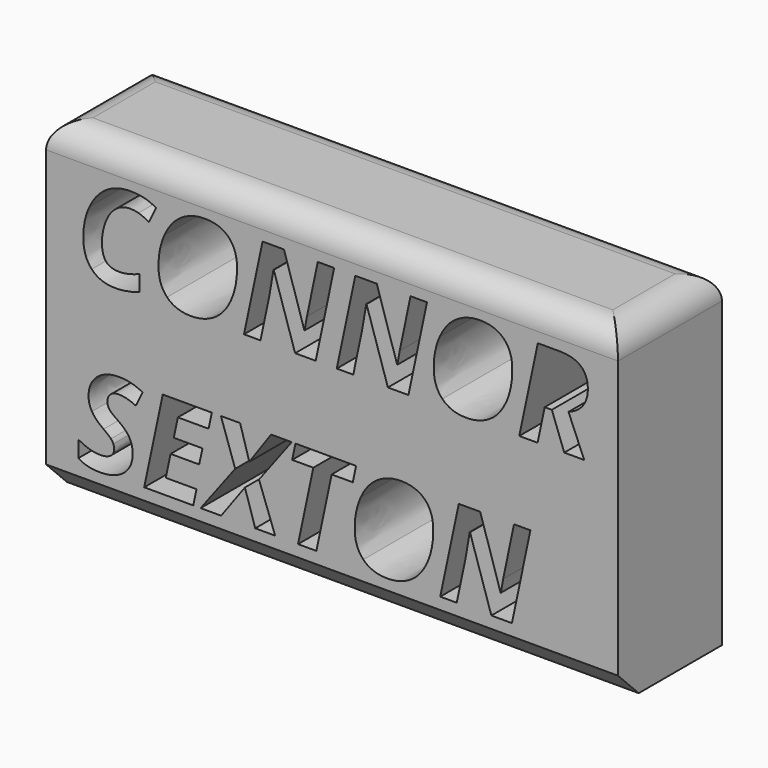
from build123d import *

# Parameters (mm, degrees)
F0_W     = 111.7530614138
F0_H     = 64.2868950963
F1_DEPTH = 25.4
F2_R     = 5.08
F3_SIZE  = 5.08


with BuildPart() as f1:
    # F0 (on Front) → F1 (new body)
    with BuildSketch(Plane.XZ):
        with Locations((-55.8765307069, 32.1434475482)):
            Rectangle(F0_W, F0_H)
        with BuildLine():
            add(Edge.make_bspline(
                [(-95.5342243518, 15.0884542018), (-94.8306232438, 13.9570636201), (-94.8306232438, 12.4447903053)],
                knots=[0, 0, 0, 1, 1, 1], degree=2))
            add(Edge.make_bspline(
                [(-94.8306232438, 12.4447903053), (-94.8306232438, 9.9943821797), (-96.5661726436, 8.5684172674)],
                knots=[0, 0, 0, 1, 1, 1], degree=2))
            add(Edge.make_bspline(
                [(-96.5661726436, 8.5684172674), (-98.3017220434, 7.1424523551), (-101.2662280453, 7.1424523551)],
                knots=[0, 0, 0, 1, 1, 1], degree=2))
            add(Edge.make_bspline(
                [(-101.2662280453, 7.1424523551), (-103.8592326621, 7.1424523551), (-105.4428042226, 8.2006684216)],
                knots=[0, 0, 0, 1, 1, 1], degree=2))
            Line((-105.4428042226, 8.2006684216), (-105.4428042226, 11.4128420135))
            add(Edge.make_bspline(
                [(-105.4428042226, 11.4128420135), (-103.1800230591, 10.1482362886), (-101.2437128098, 10.1482362886)],
                knots=[0, 0, 0, 1, 1, 1], degree=2))
            add(Edge.make_bspline(
                [(-101.2437128098, 10.1482362886), (-99.9303240748, 10.1482362886), (-99.191073844, 10.6454477383)],
                knots=[0, 0, 0, 1, 1, 1], degree=2))
            add(Edge.make_bspline(
                [(-99.191073844, 10.6454477383), (-98.4518236131, 11.142659188), (-98.4518236131, 12.0094957531)],
                knots=[0, 0, 0, 1, 1, 1], degree=2))
            add(Edge.make_bspline(
                [(-98.4518236131, 12.0094957531), (-98.4518236131, 12.5160885509), (-98.611306531, 12.896971284)],
                knots=[0, 0, 0, 1, 1, 1], degree=2))
            add(Edge.make_bspline(
                [(-98.611306531, 12.896971284), (-98.7707894488, 13.2778540172), (-99.0634875097, 13.6062012009)],
                knots=[0, 0, 0, 1, 1, 1], degree=2))
            add(Edge.make_bspline(
                [(-99.0634875097, 13.6062012009), (-99.3561855707, 13.9345483847), (-100.5157201967, 14.8013849498)],
                knots=[0, 0, 0, 1, 1, 1], degree=2))
            add(Edge.make_bspline(
                [(-100.5157201967, 14.8013849498), (-102.1368171496, 15.9646721151), (-102.7935115171, 17.1016915056)],
                knots=[0, 0, 0, 1, 1, 1], degree=2))
            add(Edge.make_bspline(
                [(-102.7935115171, 17.1016915056), (-103.4502058846, 18.2387108962), (-103.4502058846, 19.5520996312)],
                knots=[0, 0, 0, 1, 1, 1], degree=2))
            add(Edge.make_bspline(
                [(-103.4502058846, 19.5520996312), (-103.4502058846, 21.0643729461), (-102.7222132715, 22.2539278861)],
                knots=[0, 0, 0, 1, 1, 1], degree=2))
            add(Edge.make_bspline(
                [(-102.7222132715, 22.2539278861), (-101.9942206584, 23.443482826), (-100.6508116094, 24.1058060024)],
                knots=[0, 0, 0, 1, 1, 1], degree=2))
            add(Edge.make_bspline(
                [(-100.6508116094, 24.1058060024), (-99.3074025605, 24.7681291788), (-97.5624718126, 24.7681291788)],
                knots=[0, 0, 0, 1, 1, 1], degree=2))
            add(Edge.make_bspline(
                [(-97.5624718126, 24.7681291788), (-95.0182502059, 24.7681291788), (-92.9055706122, 23.6085945527)],
                knots=[0, 0, 0, 1, 1, 1], degree=2))
            Line((-92.9055706122, 23.6085945527), (-94.185186494, 20.8767459839))
            add(Edge.make_bspline(
                [(-94.185186494, 20.8767459839), (-96.0126731053, 21.743582549), (-97.5624718126, 21.743582549)],
                knots=[0, 0, 0, 1, 1, 1], degree=2))
            add(Edge.make_bspline(
                [(-97.5624718126, 21.743582549), (-98.5343794765, 21.743582549), (-99.1554247212, 21.2163507854)],
                knots=[0, 0, 0, 1, 1, 1], degree=2))
            add(Edge.make_bspline(
                [(-99.1554247212, 21.2163507854), (-99.7764699659, 20.6891190218), (-99.7764699659, 19.8222824567)],
                knots=[0, 0, 0, 1, 1, 1], degree=2))
            add(Edge.make_bspline(
                [(-99.7764699659, 19.8222824567), (-99.7764699659, 19.1055474613), (-99.3899584238, 18.5726868888)],
                knots=[0, 0, 0, 1, 1, 1], degree=2))
            add(Edge.make_bspline(
                [(-99.3899584238, 18.5726868888), (-99.0034468818, 18.0398263163), (-97.6562852937, 17.1579795943)],
                knots=[0, 0, 0, 1, 1, 1], degree=2))
            add(Edge.make_bspline(
                [(-97.6562852937, 17.1579795943), (-96.2378254599, 16.2198447836), (-95.5342243518, 15.0884542018)],
                knots=[0, 0, 0, 1, 1, 1], degree=2))
        make_face(mode=Mode.SUBTRACT)
        Polygon((-82.3609353398, 10.3808937217), (-82.9951144719, 7.3788623274), (-92.5753471588, 7.3788623274), (-88.9541467895, 24.524214128), (-79.3589039455, 24.524214128), (-79.9930830776, 21.5446979692), (-85.9971458661, 21.5446979692), (-86.7851791071, 17.7809011086), (-81.1901430961, 17.7809011086), (-81.8355798458, 14.8013849498), (-87.4268633177, 14.8013849498), (-88.3649981284, 10.3808937217), align=None, mode=Mode.SUBTRACT)
        Polygon((-70.1426675651, 16.0209602037), (-66.9980396796, 7.3788623274), (-70.881917796, 7.3788623274), (-72.8970313694, 13.7469214225), (-77.542674952, 7.3788623274), (-81.5541394026, 7.3788623274), (-74.7995687655, 16.3399260393), (-77.5877054229, 24.524214128), (-73.8351661801, 24.524214128), (-72.041452422, 18.4488530938), (-67.7860729206, 24.524214128), (-63.7520932346, 24.524214128), align=None, mode=Mode.SUBTRACT)
        Polygon((-55.9543166879, 21.4996674982), (-58.9338328467, 7.3788623274), (-62.5100027452, 7.3788623274), (-59.5304865864, 21.4996674982), (-63.6582797535, 21.4996674982), (-63.0128430037, 24.524214128), (-51.1698291533, 24.524214128), (-51.8152659031, 21.4996674982), align=None, mode=Mode.SUBTRACT)
        with BuildLine():
            add(Edge.make_bspline(
                [(-37.7301098551, 23.1057542942), (-36.0883739363, 21.4171116349), (-36.0883739363, 18.3775548482)],
                knots=[0, 0, 0, 1, 1, 1], degree=2))
            add(Edge.make_bspline(
                [(-36.0883739363, 18.3775548482), (-36.0883739363, 15.0603101575), (-37.249784832, 12.4391614964)],
                knots=[0, 0, 0, 1, 1, 1], degree=2))
            add(Edge.make_bspline(
                [(-37.249784832, 12.4391614964), (-38.4111957276, 9.8180128353), (-40.4281855707, 8.4802325952)],
                knots=[0, 0, 0, 1, 1, 1], degree=2))
            add(Edge.make_bspline(
                [(-40.4281855707, 8.4802325952), (-42.4451754137, 7.1424523551), (-45.0719528837, 7.1424523551)],
                knots=[0, 0, 0, 1, 1, 1], degree=2))
            add(Edge.make_bspline(
                [(-45.0719528837, 7.1424523551), (-48.073984278, 7.1424523551), (-49.7569981284, 8.8723729461)],
                knots=[0, 0, 0, 1, 1, 1], degree=2))
            add(Edge.make_bspline(
                [(-49.7569981284, 8.8723729461), (-51.4400119788, 10.602293537), (-51.4400119788, 13.6756231769)],
                knots=[0, 0, 0, 1, 1, 1], degree=2))
            add(Edge.make_bspline(
                [(-51.4400119788, 13.6756231769), (-51.4400119788, 16.78272567), (-50.2786010831, 19.3926167134)],
                knots=[0, 0, 0, 1, 1, 1], degree=2))
            add(Edge.make_bspline(
                [(-50.2786010831, 19.3926167134), (-49.1171901875, 22.0025077568), (-47.0758088394, 23.3984523551)],
                knots=[0, 0, 0, 1, 1, 1], degree=2))
            add(Edge.make_bspline(
                [(-47.0758088394, 23.3984523551), (-45.0344274913, 24.7943969535), (-42.3626195503, 24.7943969535)],
                knots=[0, 0, 0, 1, 1, 1], degree=2))
            add(Edge.make_bspline(
                [(-42.3626195503, 24.7943969535), (-39.3718457738, 24.7943969535), (-37.7301098551, 23.1057542942)],
                knots=[0, 0, 0, 1, 1, 1], degree=2))
        make_face(mode=Mode.SUBTRACT)
        with BuildLine():
            Line((-17.1005253675, 24.524214128), (-20.7254782761, 7.3788623274))
            Line((-20.7254782761, 7.3788623274), (-24.7369427267, 7.3788623274))
            Line((-24.7369427267, 7.3788623274), (-28.9097663648, 20.3476379507))
            Line((-28.9097663648, 20.3476379507), (-28.9810646104, 20.3476379507))
            Line((-28.9810646104, 20.3476379507), (-29.0298476205, 19.9723840264))
            add(Edge.make_bspline(
                [(-29.0298476205, 19.9723840264), (-29.4051015448, 17.4394200375), (-29.8028707045, 15.4468216995)],
                knots=[0, 0, 0, 1, 1, 1], degree=2))
            Line((-29.8028707045, 15.4468216995), (-31.5027709816, 7.3788623274))
            Line((-31.5027709816, 7.3788623274), (-34.7262021912, 7.3788623274))
            Line((-34.7262021912, 7.3788623274), (-31.1050018218, 24.524214128))
            Line((-31.1050018218, 24.524214128), (-26.9171680268, 24.524214128))
            Line((-26.9171680268, 24.524214128), (-22.9319713509, 11.8931670366))
            Line((-22.9319713509, 11.8931670366), (-22.8831883407, 11.8931670366))
            add(Edge.make_bspline(
                [(-22.8831883407, 11.8931670366), (-22.7443443888, 12.7862713764), (-22.4272548227, 14.4392649128)],
                knots=[0, 0, 0, 1, 1, 1], degree=2))
            add(Edge.make_bspline(
                [(-22.4272548227, 14.4392649128), (-22.1101652567, 16.0922584493), (-20.3164514986, 24.524214128)],
                knots=[0, 0, 0, 1, 1, 1], degree=2))
            Line((-20.3164514986, 24.524214128), (-17.1005253675, 24.524214128))
        make_face(mode=Mode.SUBTRACT)
        with BuildLine():
            add(Edge.make_bspline(
                [(-93.7029852013, 54.2067995389), (-94.5116574081, 54.4281993542), (-95.3109482669, 54.4281993542)],
                knots=[0, 0, 0, 1, 1, 1], degree=2))
            add(Edge.make_bspline(
                [(-95.3109482669, 54.4281993542), (-96.8569944349, 54.4281993542), (-98.0953323851, 53.4788069258)],
                knots=[0, 0, 0, 1, 1, 1], degree=2))
            add(Edge.make_bspline(
                [(-98.0953323851, 53.4788069258), (-99.3336703352, 52.5294144973), (-100.0841781838, 50.6831651898)],
                knots=[0, 0, 0, 1, 1, 1], degree=2))
            add(Edge.make_bspline(
                [(-100.0841781838, 50.6831651898), (-100.8346860323, 48.8369158824), (-100.8346860323, 46.7129786709)],
                knots=[0, 0, 0, 1, 1, 1], degree=2))
            add(Edge.make_bspline(
                [(-100.8346860323, 46.7129786709), (-100.8346860323, 44.7541531862), (-100.0316426344, 43.8047607577)],
                knots=[0, 0, 0, 1, 1, 1], degree=2))
            add(Edge.make_bspline(
                [(-100.0316426344, 43.8047607577), (-99.2285992364, 42.8553683293), (-97.4686583315, 42.8553683293)],
                knots=[0, 0, 0, 1, 1, 1], degree=2))
            add(Edge.make_bspline(
                [(-97.4686583315, 42.8553683293), (-95.7575004368, 42.8553683293), (-93.5059768911, 43.7597302868)],
                knots=[0, 0, 0, 1, 1, 1], degree=2))
            Line((-93.5059768911, 43.7597302868), (-93.5059768911, 40.7089158824))
            add(Edge.make_bspline(
                [(-93.5059768911, 40.7089158824), (-95.8363037609, 39.8045539248), (-98.1966509446, 39.8045539248)],
                knots=[0, 0, 0, 1, 1, 1], degree=2))
            add(Edge.make_bspline(
                [(-98.1966509446, 39.8045539248), (-101.1724145642, 39.8045539248), (-102.8272843703, 41.5588660209)],
                knots=[0, 0, 0, 1, 1, 1], degree=2))
            add(Edge.make_bspline(
                [(-102.8272843703, 41.5588660209), (-104.4821541764, 43.3131781169), (-104.4821541764, 46.5253517088)],
                knots=[0, 0, 0, 1, 1, 1], degree=2))
            add(Edge.make_bspline(
                [(-104.4821541764, 46.5253517088), (-104.4821541764, 49.5986813487), (-103.2625789225, 52.184180887)],
                knots=[0, 0, 0, 1, 1, 1], degree=2))
            add(Edge.make_bspline(
                [(-103.2625789225, 52.184180887), (-102.0430036685, 54.7696804253), (-100.0016223204, 56.1130894742)],
                knots=[0, 0, 0, 1, 1, 1], degree=2))
            add(Edge.make_bspline(
                [(-100.0016223204, 56.1130894742), (-97.9602409723, 57.4564985232), (-95.3109482669, 57.4564985232)],
                knots=[0, 0, 0, 1, 1, 1], degree=2))
            add(Edge.make_bspline(
                [(-95.3109482669, 57.4564985232), (-93.8437054229, 57.4564985232), (-92.7066860323, 57.1919445066)],
                knots=[0, 0, 0, 1, 1, 1], degree=2))
            add(Edge.make_bspline(
                [(-92.7066860323, 57.1919445066), (-91.5696666418, 56.9273904899), (-90.2675355245, 56.2256656515)],
                knots=[0, 0, 0, 1, 1, 1], degree=2))
            Line((-90.2675355245, 56.2256656515), (-91.6522225051, 53.2911799636))
            add(Edge.make_bspline(
                [(-91.6522225051, 53.2911799636), (-92.8943129945, 53.9853997235), (-93.7029852013, 54.2067995389)],
                knots=[0, 0, 0, 1, 1, 1], degree=2))
        make_face(mode=Mode.SUBTRACT)
        with BuildLine():
            add(Edge.make_bspline(
                [(-76.0773083777, 55.7678558639), (-74.4355724589, 54.0792132046), (-74.4355724589, 51.0396564179)],
                knots=[0, 0, 0, 1, 1, 1], degree=2))
            add(Edge.make_bspline(
                [(-74.4355724589, 51.0396564179), (-74.4355724589, 47.7224117272), (-75.5969833546, 45.1012630661)],
                knots=[0, 0, 0, 1, 1, 1], degree=2))
            add(Edge.make_bspline(
                [(-75.5969833546, 45.1012630661), (-76.7583942503, 42.480114405), (-78.7753840933, 41.1423341649)],
                knots=[0, 0, 0, 1, 1, 1], degree=2))
            add(Edge.make_bspline(
                [(-78.7753840933, 41.1423341649), (-80.7923739363, 39.8045539248), (-83.4191514063, 39.8045539248)],
                knots=[0, 0, 0, 1, 1, 1], degree=2))
            add(Edge.make_bspline(
                [(-83.4191514063, 39.8045539248), (-86.4211828006, 39.8045539248), (-88.104196651, 41.5344745158)],
                knots=[0, 0, 0, 1, 1, 1], degree=2))
            add(Edge.make_bspline(
                [(-88.104196651, 41.5344745158), (-89.7872105014, 43.2643951067), (-89.7872105014, 46.3377247466)],
                knots=[0, 0, 0, 1, 1, 1], degree=2))
            add(Edge.make_bspline(
                [(-89.7872105014, 46.3377247466), (-89.7872105014, 49.4448272397), (-88.6257996057, 52.0547182831)],
                knots=[0, 0, 0, 1, 1, 1], degree=2))
            add(Edge.make_bspline(
                [(-88.6257996057, 52.0547182831), (-87.4643887101, 54.6646093265), (-85.423007362, 56.0605539248)],
                knots=[0, 0, 0, 1, 1, 1], degree=2))
            add(Edge.make_bspline(
                [(-85.423007362, 56.0605539248), (-83.3816260139, 57.4564985232), (-80.709818073, 57.4564985232)],
                knots=[0, 0, 0, 1, 1, 1], degree=2))
            add(Edge.make_bspline(
                [(-80.709818073, 57.4564985232), (-77.7190442964, 57.4564985232), (-76.0773083777, 55.7678558639)],
                knots=[0, 0, 0, 1, 1, 1], degree=2))
        make_face(mode=Mode.SUBTRACT)
        with BuildLine():
            Line((-55.4477238901, 57.1863156977), (-59.0726767987, 40.0409638971))
            Line((-59.0726767987, 40.0409638971), (-63.0841412493, 40.0409638971))
            Line((-63.0841412493, 40.0409638971), (-67.2569648874, 53.0097395204))
            Line((-67.2569648874, 53.0097395204), (-67.328263133, 53.0097395204))
            Line((-67.328263133, 53.0097395204), (-67.3770461431, 52.6344855961))
            add(Edge.make_bspline(
                [(-67.3770461431, 52.6344855961), (-67.7523000674, 50.1015216072), (-68.1500692272, 48.1089232693)],
                knots=[0, 0, 0, 1, 1, 1], degree=2))
            Line((-68.1500692272, 48.1089232693), (-69.8499695042, 40.0409638971))
            Line((-69.8499695042, 40.0409638971), (-73.0734007138, 40.0409638971))
            Line((-73.0734007138, 40.0409638971), (-69.4522003444, 57.1863156977))
            Line((-69.4522003444, 57.1863156977), (-65.2643665494, 57.1863156977))
            Line((-65.2643665494, 57.1863156977), (-61.2791698735, 44.5552686063))
            Line((-61.2791698735, 44.5552686063), (-61.2303868634, 44.5552686063))
            add(Edge.make_bspline(
                [(-61.2303868634, 44.5552686063), (-61.0915429114, 45.4483729461), (-60.7744533454, 47.1013664826)],
                knots=[0, 0, 0, 1, 1, 1], degree=2))
            add(Edge.make_bspline(
                [(-60.7744533454, 47.1013664826), (-60.4573637793, 48.754360019), (-58.6636500213, 57.1863156977)],
                knots=[0, 0, 0, 1, 1, 1], degree=2))
            Line((-58.6636500213, 57.1863156977), (-55.4477238901, 57.1863156977))
        make_face(mode=Mode.SUBTRACT)
        with BuildLine():
            Line((-37.319206808, 57.1863156977), (-40.9441597166, 40.0409638971))
            Line((-40.9441597166, 40.0409638971), (-44.9556241672, 40.0409638971))
            Line((-44.9556241672, 40.0409638971), (-49.1284478052, 53.0097395204))
            Line((-49.1284478052, 53.0097395204), (-49.1997460508, 53.0097395204))
            Line((-49.1997460508, 53.0097395204), (-49.248529061, 52.6344855961))
            add(Edge.make_bspline(
                [(-49.248529061, 52.6344855961), (-49.6237829853, 50.1015216072), (-50.021552145, 48.1089232693)],
                knots=[0, 0, 0, 1, 1, 1], degree=2))
            Line((-50.021552145, 48.1089232693), (-51.721452422, 40.0409638971))
            Line((-51.721452422, 40.0409638971), (-54.9448836316, 40.0409638971))
            Line((-54.9448836316, 40.0409638971), (-51.3236832623, 57.1863156977))
            Line((-51.3236832623, 57.1863156977), (-47.1358494672, 57.1863156977))
            Line((-47.1358494672, 57.1863156977), (-43.1506527913, 44.5552686063))
            Line((-43.1506527913, 44.5552686063), (-43.1018697812, 44.5552686063))
            add(Edge.make_bspline(
                [(-43.1018697812, 44.5552686063), (-42.9630258292, 45.4483729461), (-42.6459362632, 47.1013664826)],
                knots=[0, 0, 0, 1, 1, 1], degree=2))
            add(Edge.make_bspline(
                [(-42.6459362632, 47.1013664826), (-42.3288466972, 48.754360019), (-40.5351329391, 57.1863156977)],
                knots=[0, 0, 0, 1, 1, 1], degree=2))
            Line((-40.5351329391, 57.1863156977), (-37.319206808, 57.1863156977))
        make_face(mode=Mode.SUBTRACT)
        with BuildLine():
            add(Edge.make_bspline(
                [(-22.2884108708, 55.7678558639), (-20.646674952, 54.0792132046), (-20.646674952, 51.0396564179)],
                knots=[0, 0, 0, 1, 1, 1], degree=2))
            add(Edge.make_bspline(
                [(-20.646674952, 51.0396564179), (-20.646674952, 47.7224117272), (-21.8080858477, 45.1012630661)],
                knots=[0, 0, 0, 1, 1, 1], degree=2))
            add(Edge.make_bspline(
                [(-21.8080858477, 45.1012630661), (-22.9694967433, 42.480114405), (-24.9864865864, 41.1423341649)],
                knots=[0, 0, 0, 1, 1, 1], degree=2))
            add(Edge.make_bspline(
                [(-24.9864865864, 41.1423341649), (-27.0034764294, 39.8045539248), (-29.6302538994, 39.8045539248)],
                knots=[0, 0, 0, 1, 1, 1], degree=2))
            add(Edge.make_bspline(
                [(-29.6302538994, 39.8045539248), (-32.6322852937, 39.8045539248), (-34.3152991441, 41.5344745158)],
                knots=[0, 0, 0, 1, 1, 1], degree=2))
            add(Edge.make_bspline(
                [(-34.3152991441, 41.5344745158), (-35.9983129945, 43.2643951067), (-35.9983129945, 46.3377247466)],
                knots=[0, 0, 0, 1, 1, 1], degree=2))
            add(Edge.make_bspline(
                [(-35.9983129945, 46.3377247466), (-35.9983129945, 49.4448272397), (-34.8369020988, 52.0547182831)],
                knots=[0, 0, 0, 1, 1, 1], degree=2))
            add(Edge.make_bspline(
                [(-34.8369020988, 52.0547182831), (-33.6754912032, 54.6646093265), (-31.6341098551, 56.0605539248)],
                knots=[0, 0, 0, 1, 1, 1], degree=2))
            add(Edge.make_bspline(
                [(-31.6341098551, 56.0605539248), (-29.5927285069, 57.4564985232), (-26.920920566, 57.4564985232)],
                knots=[0, 0, 0, 1, 1, 1], degree=2))
            add(Edge.make_bspline(
                [(-26.920920566, 57.4564985232), (-23.9301467895, 57.4564985232), (-22.2884108708, 55.7678558639)],
                knots=[0, 0, 0, 1, 1, 1], degree=2))
        make_face(mode=Mode.SUBTRACT)
        with BuildLine():
            Line((-12.9164441118, 46.6191651898), (-14.3123887101, 46.6191651898))
            Line((-14.3123887101, 46.6191651898), (-15.7083333084, 40.0409638971))
            Line((-15.7083333084, 40.0409638971), (-19.2845032069, 40.0409638971))
            Line((-19.2845032069, 40.0409638971), (-15.6633028375, 57.1863156977))
            Line((-15.6633028375, 57.1863156977), (-11.452953807, 57.1863156977))
            add(Edge.make_bspline(
                [(-11.452953807, 57.1863156977), (-8.6723222281, 57.1863156977), (-7.2763776298, 55.9892556792)],
                knots=[0, 0, 0, 1, 1, 1], degree=2))
            add(Edge.make_bspline(
                [(-7.2763776298, 55.9892556792), (-5.8804330314, 54.7921956608), (-5.8804330314, 52.4843840264)],
                knots=[0, 0, 0, 1, 1, 1], degree=2))
            add(Edge.make_bspline(
                [(-5.8804330314, 52.4843840264), (-5.8804330314, 50.6306296404), (-6.8542169649, 49.3003544789)],
                knots=[0, 0, 0, 1, 1, 1], degree=2))
            add(Edge.make_bspline(
                [(-6.8542169649, 49.3003544789), (-7.8280008985, 47.9700793173), (-9.659240049, 47.3246425675)],
                knots=[0, 0, 0, 1, 1, 1], degree=2))
            Line((-9.659240049, 47.3246425675), (-6.5971680268, 40.0409638971))
            Line((-6.5971680268, 40.0409638971), (-10.4923037609, 40.0409638971))
            Line((-10.4923037609, 40.0409638971), (-12.9164441118, 46.6191651898))
        make_face(mode=Mode.SUBTRACT)
    extrude(amount=F1_DEPTH)

    # F2
    f2_edges = [f1.edges().sort_by_distance(p)[0] for p in [
        (-55.876531, -25.4, 64.286895),
        (-55.876531, 0, 64.286895),
        (0, -12.7, 64.286895),
        (-111.753061, -12.7, 64.286895),
    ]]
    fillet(f2_edges, radius=F2_R)

    # F3
    f3_edges = [f1.edges().sort_by_distance(p)[0] for p in [
        (-55.876531, -25.4, 0),
    ]]
    chamfer(f3_edges, length=F3_SIZE)


solid = f1.part
